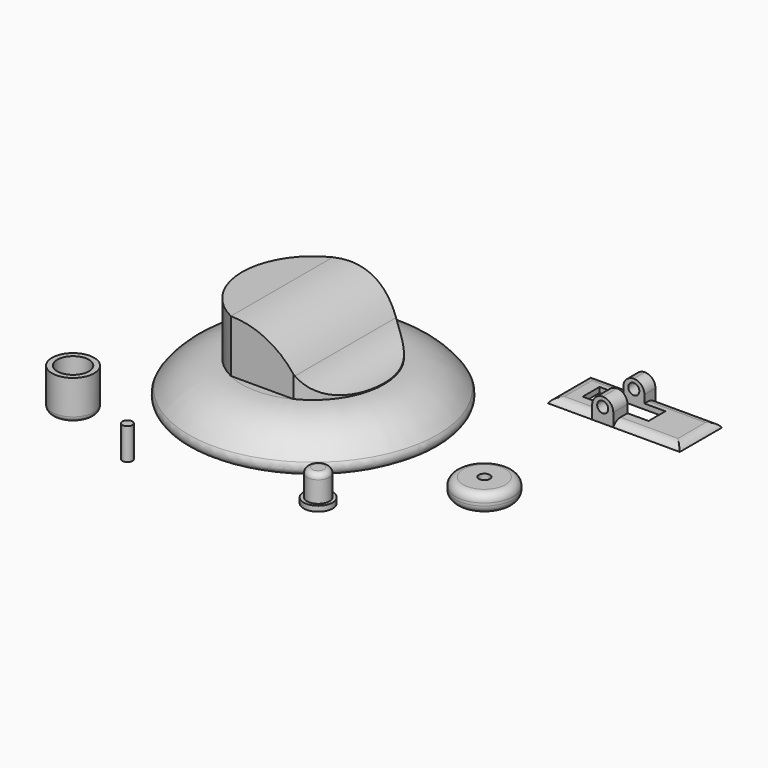
from build123d import *

# Parameters (mm, degrees)
F0_R          = 63.5
F1_DEPTH      = 19.05
F3_R          = 3.81
F4_R          = 34.2243208574
F5_DEPTH      = 25.4
F6_R          = 23.0273094471
F7_DEPTH      = 60.7519101096
F8_DEPTH      = 71.374
F9_R          = 38.1
F10_R         = 7.62
F10_R_2       = 5.715
F11_DEPTH     = 1.27
F10_R_3       = 10.16
F12_DEPTH     = 19.05
F13_R         = 2.54
F14_R         = 6.985
F15_DEPTH     = 2.54
F16_R         = 5.3975
F17_DEPTH     = 12.7
F18_R         = 2.54
F19_W         = 30.2823996797
F19_H         = 4.1530619248
F20_DEPTH     = 25.4
F21_W         = 63.5
F21_H         = 25.4
F21_W_2       = 31.75
F21_H_2       = 10.16
F22_DEPTH     = 2.54
F23_W         = 10.16
F23_H         = 8.5772957325
F23_H_2       = 6.6627042675
F24_DEPTH     = 8.89
F25_R         = 5.08
F26_R         = 5.07999
F28_R         = 2.667
F29_DEPTH     = 150.114
F30_T1_DEPTH  = 43.0515242213
F30_T3_DEPTH  = 47.3970452561
F30_T5_DEPTH  = 32.2855210348
F30_T10_DEPTH = 54.0500468494
F30_T15_DEPTH = 54.0500468494
F30_T20_DEPTH = 43.2840436629
F30_T25_DEPTH = 43.2840436629
F21_R         = 13.97
F31_DEPTH     = 8.89
F32_R         = 3.81
F33_R         = 2.667
F34_DEPTH     = 29.464
F35_R         = 2.413
F36_DEPTH     = 15.24


# Not quite as in the source:
# - a fillet or chamfer that OpenCascade refuses, or shapes differently, is made with other operations: its cross-section is extruded or revolved along the edge and cut away or added
# - a fillet or chamfer is up to 0.001 mm smaller than in the source, because OpenCascade refuses the exact size


with BuildPart() as f1:
    # F0 (on Top) → F1 (new body)
    with BuildSketch(Plane.XY):
        Circle(F0_R)
    extrude(amount=F1_DEPTH)

    # F2: fillet of radius 31.75 on 1 edges, made by hand

    # F2_s1 → F2_t2 (revolve, cut)
    with BuildSketch(Plane.XZ):
        with BuildLine():
            ThreePointArc((63.5, 0), (51.7908355378, 13.8639558425), (34.400644337, 19.05))
            Line((34.400644337, 19.05), (63.5, 19.05))
            Line((63.5, 19.05), (63.5, 0))
        make_face()
    revolve(axis=Axis((0, 0, 19.05), (0, 0, 1)), mode=Mode.SUBTRACT)

    # F3
    f3_edges = [f1.edges().sort_by_distance(p)[0] for p in [
        (-63.5, 0, 0),
    ]]
    fillet(f3_edges, radius=F3_R)

    # F4 (on face) → F5 (join)
    with BuildSketch(Plane.XY.offset(19.05)):
        Circle(F4_R)
    extrude(amount=F5_DEPTH)

    # F6 (on Front) → F7 (cut, through all)
    with BuildSketch(Plane.XZ):
        with Locations((34.1903194785, 42.5634607673)):
            Circle(F6_R)
    extrude(amount=F7_DEPTH, mode=Mode.SUBTRACT)

    # F6 (on Front) → F8 (cut)
    with BuildSketch(Plane.XZ):
        with Locations((34.1903194785, 42.5634607673)):
            Circle(F6_R)
    extrude(amount=-F8_DEPTH, mode=Mode.SUBTRACT)

    # F9
    f9_edges = [f1.edges().sort_by_distance(p)[0] for p in [
        (11.240419, 0, 44.45),
    ]]
    fillet(f9_edges, radius=F9_R)

    # F19 (on face) → F20 (cut)
    with BuildSketch(Plane.XY.offset(44.45)):
        with Locations((0.085877689, -32.8115502902)):
            Rectangle(F19_W, F19_H)
    extrude(amount=-F20_DEPTH, mode=Mode.SUBTRACT)


with BuildPart() as f11:
    # F10 (on Top) → F11 (new body)
    with BuildSketch(Plane.XY):
        with Locations((-66.7525306344, -61.1704364419)):
            Circle(F10_R)
        with Locations((-66.7525306344, -61.1704364419)):
            Circle(F10_R_2, mode=Mode.SUBTRACT)
    extrude(amount=F11_DEPTH)

    # F10 (on Top) → F12 (join)
    with BuildSketch(Plane.XY):
        with Locations((-66.7525306344, -61.1704364419)):
            Circle(F10_R_3)
        with Locations((-66.7525306344, -61.1704364419)):
            Circle(F10_R, mode=Mode.SUBTRACT)
    extrude(amount=F12_DEPTH)

    # F13
    f13_edges = [f11.edges().sort_by_distance(p)[0] for p in [
        (-76.912531, -61.170436, 0),
    ]]
    fillet(f13_edges, radius=F13_R)


with BuildPart() as f15:
    # F14 (on Top) → F15 (new body)
    with BuildSketch(Plane.XY):
        with Locations((52.5529012084, -62.5889375806)):
            Circle(F14_R)
    extrude(amount=F15_DEPTH)

    # F16 (on face) → F17 (join)
    with BuildSketch(Plane.XY.offset(2.54)):
        with Locations((52.5529012084, -62.5889375806)):
            Circle(F16_R)
    extrude(amount=F17_DEPTH)

    # F18
    f18_edges = [f15.edges().sort_by_distance(p)[0] for p in [
        (47.155401, -62.588938, 15.24),
    ]]
    fillet(f18_edges, radius=F18_R)


with BuildPart() as f22:
    # F21 (on Top) → F22 (new body)
    with BuildSketch(Plane.XY):
        with Locations((100.9996779405, 67.7282363176)):
            Rectangle(F21_W, F21_H)
        with Locations((94.9586960077, 68.6855320501)):
            Rectangle(F21_W_2, F21_H_2, mode=Mode.SUBTRACT)
    extrude(amount=F22_DEPTH)

    # F23 (on face) → F24 (join)
    with BuildSketch(Plane.XY.offset(2.54)):
        with Locations((95.6166763473, 59.3168841839)):
            Rectangle(F23_W, F23_H)
        with Locations((95.6166763473, 77.0968841839)):
            Rectangle(F23_W, F23_H_2)
    extrude(amount=F24_DEPTH)

    # F25
    f25_edges = [f22.edges().sort_by_distance(p)[0] for p in [
        (90.536676, 77.096884, 11.43),
        (90.536676, 59.316884, 11.43),
    ]]
    fillet(f25_edges, radius=F25_R)

    # F26 (radius 5.08 in the source; OpenCascade refuses exactly that, so slightly less here)
    f26_edges = [f22.edges().sort_by_distance(p)[0] for p in [
        (100.696676, 59.316884, 11.43),
        (100.696676, 77.096884, 11.43),
    ]]
    fillet(f26_edges, radius=F26_R)

    # F28 (on face) → F29 (cut)
    with BuildSketch(Plane.XZ.offset(-55.0282363176)):
        with Locations((95.6014543772, 6.9776163436)):
            Circle(F28_R)
    extrude(amount=-F29_DEPTH, mode=Mode.SUBTRACT)

    # F30: fillet of radius 5.08 on 6 edges, made by hand

    # F30_s2 → F30_t1 (cut)
    with BuildSketch(Plane.YZ.offset(100.6966763473)):
        with BuildLine():
            ThreePointArc((80.4282363176, 0), (78.5688272664, 1.8594090512), (76.0288272664, 2.54))
            Line((76.0288272664, 2.54), (80.4282363176, 2.54))
            Line((80.4282363176, 2.54), (80.4282363176, 0))
        make_face()
        with BuildLine():
            ThreePointArc((59.4276453689, 2.54), (56.8876453689, 1.8594090512), (55.0282363176, 0))
            Line((55.0282363176, 0), (55.0282363176, 2.54))
            Line((55.0282363176, 2.54), (59.4276453689, 2.54))
        make_face()
    extrude(amount=F30_T1_DEPTH, mode=Mode.SUBTRACT)

    # F30_s4 → F30_t3 (cut)
    with BuildSketch(Plane.XZ.offset(-91.4267589457)):
        with BuildLine():
            ThreePointArc((128.3502688893, 2.54), (130.8902688893, 1.8594090512), (132.7496779405, 0))
            Line((132.7496779405, 0), (132.7496779405, 2.54))
            Line((132.7496779405, 2.54), (128.3502688893, 2.54))
        make_face()
        with BuildLine():
            ThreePointArc((73.6490869917, 2.54), (71.1090869917, 1.8594090512), (69.2496779405, 0))
            Line((69.2496779405, 0), (69.2496779405, 2.54))
            Line((69.2496779405, 2.54), (73.6490869917, 2.54))
        make_face()
    extrude(amount=F30_T3_DEPTH, mode=Mode.SUBTRACT)

    # F30_s6 → F30_t5 (cut)
    with BuildSketch(Plane.YZ.offset(58.2511553124)):
        with BuildLine():
            ThreePointArc((80.4282363176, 0), (78.5688272664, 1.8594090512), (76.0288272664, 2.54))
            Line((76.0288272664, 2.54), (80.4282363176, 2.54))
            Line((80.4282363176, 2.54), (80.4282363176, 0))
        make_face()
        with BuildLine():
            ThreePointArc((59.4276453689, 2.54), (56.8876453689, 1.8594090512), (55.0282363176, 0))
            Line((55.0282363176, 0), (55.0282363176, 2.54))
            Line((55.0282363176, 2.54), (59.4276453689, 2.54))
        make_face()
    extrude(amount=F30_T5_DEPTH, mode=Mode.SUBTRACT)


with BuildPart() as f30_tool8:
    # F30_s9 → F30_t10 (new body)
    with BuildSketch(Plane.YZ.offset(143.7482005686)):
        with BuildLine():
            ThreePointArc((80.4282363176, 0), (78.5688272664, 1.8594090512), (76.0288272664, 2.54))
            Line((76.0288272664, 2.54), (80.4282363176, 2.54))
            Line((80.4282363176, 2.54), (80.4282363176, 0))
        make_face()
    extrude(amount=-F30_T10_DEPTH)

    split(bisect_by=Plane.YZ.offset(90.5366763473), keep=Keep.BOTTOM)


with BuildPart() as f22_1:
    add(f22.part)

    # F30_t7: cut F30_tool8
    add(f30_tool8.part, mode=Mode.SUBTRACT)


with BuildPart() as f30_tool13:
    # F30_s14 → F30_t15 (new body)
    with BuildSketch(Plane.YZ.offset(89.6981537192)):
        with BuildLine():
            ThreePointArc((59.4276453689, 2.54), (56.8876453689, 1.8594090512), (55.0282363176, 0))
            Line((55.0282363176, 0), (55.0282363176, 2.54))
            Line((55.0282363176, 2.54), (59.4276453689, 2.54))
        make_face()
    extrude(amount=F30_T15_DEPTH)

    split(bisect_by=Plane.YZ.offset(90.5366763473), keep=Keep.BOTTOM)


with BuildPart() as f22_2:
    add(f22_1.part)

    # F30_t12: cut F30_tool13
    add(f30_tool13.part, mode=Mode.SUBTRACT)


with BuildPart() as f30_tool18:
    # F30_s19 → F30_t20 (new body)
    with BuildSketch(Plane.YZ.offset(101.5351989753)):
        with BuildLine():
            ThreePointArc((80.4282363176, 0), (78.5688272664, 1.8594090512), (76.0288272664, 2.54))
            Line((76.0288272664, 2.54), (80.4282363176, 2.54))
            Line((80.4282363176, 2.54), (80.4282363176, 0))
        make_face()
    extrude(amount=-F30_T20_DEPTH)

    split(bisect_by=Plane.YZ.offset(100.6966763473), keep=Keep.TOP)


with BuildPart() as f22_3:
    add(f22_2.part)

    # F30_t17: cut F30_tool18
    add(f30_tool18.part, mode=Mode.SUBTRACT)


with BuildPart() as f30_tool23:
    # F30_s24 → F30_t25 (new body)
    with BuildSketch(Plane.YZ.offset(58.2511553124)):
        with BuildLine():
            ThreePointArc((59.4276453689, 2.54), (56.8876453689, 1.8594090512), (55.0282363176, 0))
            Line((55.0282363176, 0), (55.0282363176, 2.54))
            Line((55.0282363176, 2.54), (59.4276453689, 2.54))
        make_face()
    extrude(amount=F30_T25_DEPTH)

    split(bisect_by=Plane.YZ.offset(100.6966763473), keep=Keep.TOP)


with BuildPart() as f22_4:
    add(f22_3.part)

    # F30_t22: cut F30_tool23
    add(f30_tool23.part, mode=Mode.SUBTRACT)


with BuildPart() as f31:
    # F21 (on Top) → F31 (new body)
    with BuildSketch(Plane.XY):
        with Locations((98.6744686961, -20.1166216284)):
            Circle(F21_R)
    extrude(amount=F31_DEPTH)

    # F32
    f32_edges = [f31.edges().sort_by_distance(p)[0] for p in [
        (84.704469, -20.116622, 0),
        (84.704469, -20.116622, 8.89),
    ]]
    fillet(f32_edges, radius=F32_R)

    # F33 (on face) → F34 (cut)
    with BuildSketch(Plane.XY.offset(8.89)):
        with Locations((98.6744686961, -20.1166216284)):
            Circle(F33_R)
    extrude(amount=-F34_DEPTH, mode=Mode.SUBTRACT)


with BuildPart() as f36:
    # F35 (on Top) → F36 (new body)
    with BuildSketch(Plane.XY):
        with Locations((-25.9607546031, -79.4184356928)):
            Circle(F35_R)
    extrude(amount=F36_DEPTH)


solid = Compound([f1.part, f11.part, f15.part, f22_4.part, f31.part, f36.part])
